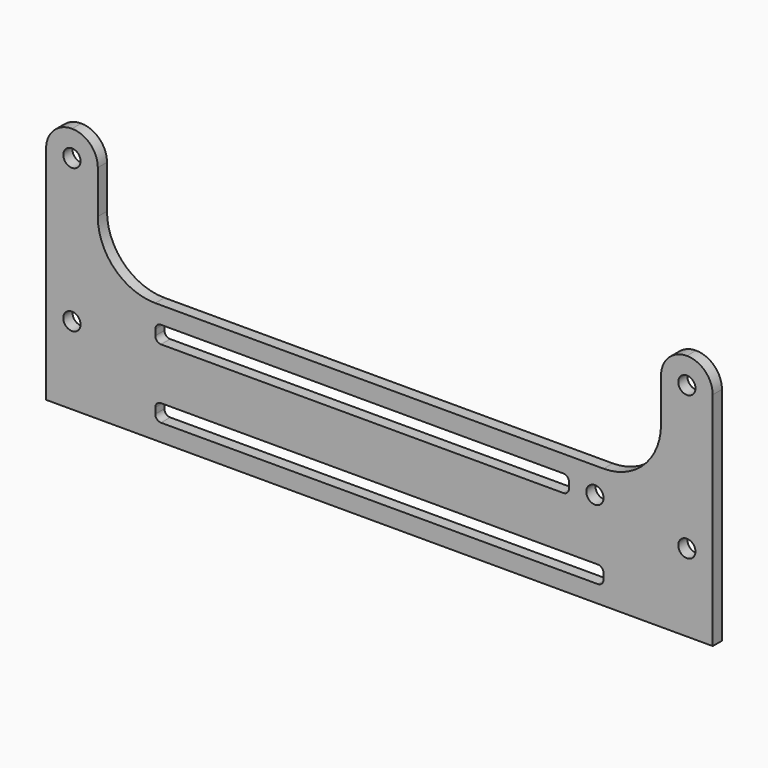
from build123d import *

# Parameters (mm, degrees)
F0_W     = 84
F0_H     = 21
F0_W_2   = 78
F0_H_2   = 3
F0_W_3   = 72
F0_R     = 1.5
F1_DEPTH = 2
F2_R     = 1
F3_R     = 1.5
F4_DEPTH = 2
F5_R     = 10
F6_R     = 4.49999


# Not quite as in the source:
# - a fillet or chamfer is up to 0.001 mm smaller than in the source, because OpenCascade refuses the exact size


with BuildPart() as f1:
    # F0 (on Front) → F1 (new body)
    with BuildSketch(Plane.XZ):
        Rectangle(F0_W, F0_H)
        with Locations((0, -6)):
            Rectangle(F0_W_2, F0_H_2, mode=Mode.SUBTRACT)
        with Locations((-3, 6)):
            Rectangle(F0_W_3, F0_H_2, mode=Mode.SUBTRACT)
        with Locations((37.5, 6)):
            Circle(F0_R, mode=Mode.SUBTRACT)
    extrude(amount=F1_DEPTH)

    # F2
    f2_edges = [f1.edges().sort_by_distance(p)[0] for p in [
        (-39, -1, 7.5),
        (-39, -1, -4.5),
        (-39, -1, 4.5),
        (-39, -1, -7.5),
        (33, -1, 7.5),
        (39, -1, -4.5),
        (39, -1, -7.5),
        (33, -1, 4.5),
    ]]
    fillet(f2_edges, radius=F2_R)

    # F3 (on face) → F4 (join)
    with BuildSketch(Plane.XZ.offset(2)):
        Polygon((-42, -10.5), (-42, 0), (-42, 10.5), (-49, 10.5), (-49, 32.5), (-58, 32.5), (-58, -10.5), align=None)
        with Locations((-53.5, 3)):
            Circle(F3_R, mode=Mode.SUBTRACT)
        with Locations((-53.5, 28)):
            Circle(F3_R, mode=Mode.SUBTRACT)
        Polygon((42, 10.5), (42, 0), (42, -10.5), (58, -10.5), (58, 32.5), (49, 32.5), (49, 10.5), align=None)
        with Locations((53.5, 3)):
            Circle(F3_R, mode=Mode.SUBTRACT)
        with Locations((53.5, 28)):
            Circle(F3_R, mode=Mode.SUBTRACT)
    extrude(amount=-F4_DEPTH)

    # F5
    f5_edges = [f1.edges().sort_by_distance(p)[0] for p in [
        (-49, -1, 10.5),
        (49, -1, 10.5),
    ]]
    fillet(f5_edges, radius=F5_R)

    # F6 (radius 4.5 in the source; OpenCascade refuses exactly that, so slightly less here)
    f6_edges = [f1.edges().sort_by_distance(p)[0] for p in [
        (-49, -1, 32.5),
        (-58, -1, 32.5),
        (58, -1, 32.5),
        (49, -1, 32.5),
    ]]
    fillet(f6_edges, radius=F6_R)


solid = f1.part
